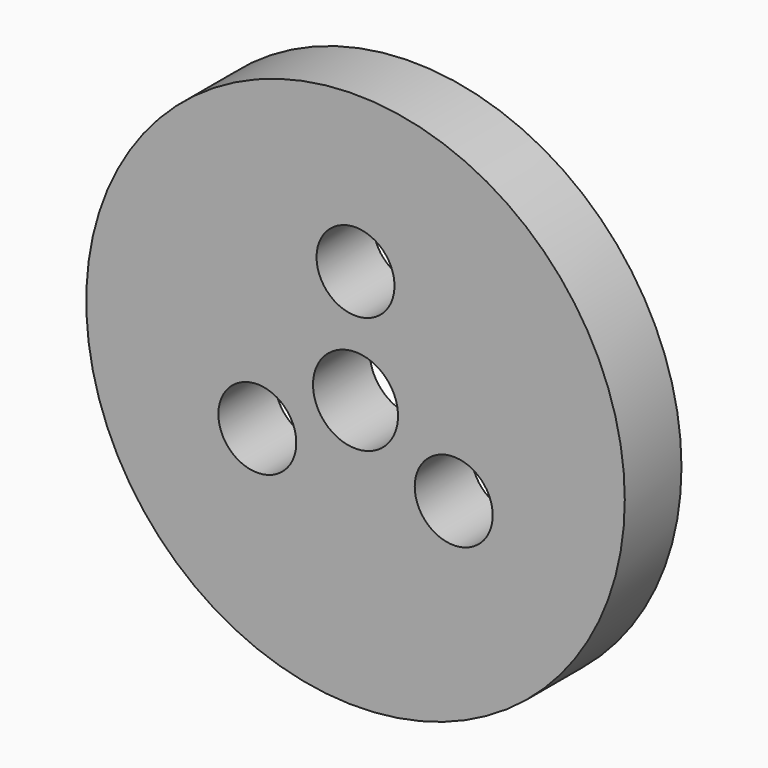
from build123d import *

# Parameters (mm, degrees)
F0_R     = 19
F1_DEPTH = 5
F4_D     = 5.5
F6_D     = 6


# Not quite as in the source:
# - a feature names something its author has since deleted; it is built from what else it names


with BuildPart() as f1:
    # F0 (on Front) → F1 (new body)
    with BuildSketch(Plane.XZ):
        Circle(F0_R)
    extrude(amount=F1_DEPTH)

    # F4 (through all)
    with Locations(Plane.XZ.offset(5)):
        with Locations((-6.9282032303, -4), (0, 8), (6.9282032303, -4)):
            Hole(F4_D / 2)

    # F6 (through all)
    with Locations(Plane.XZ.offset(5)):
        with Locations((0, 0)):
            Hole(F6_D / 2)


solid = f1.part
